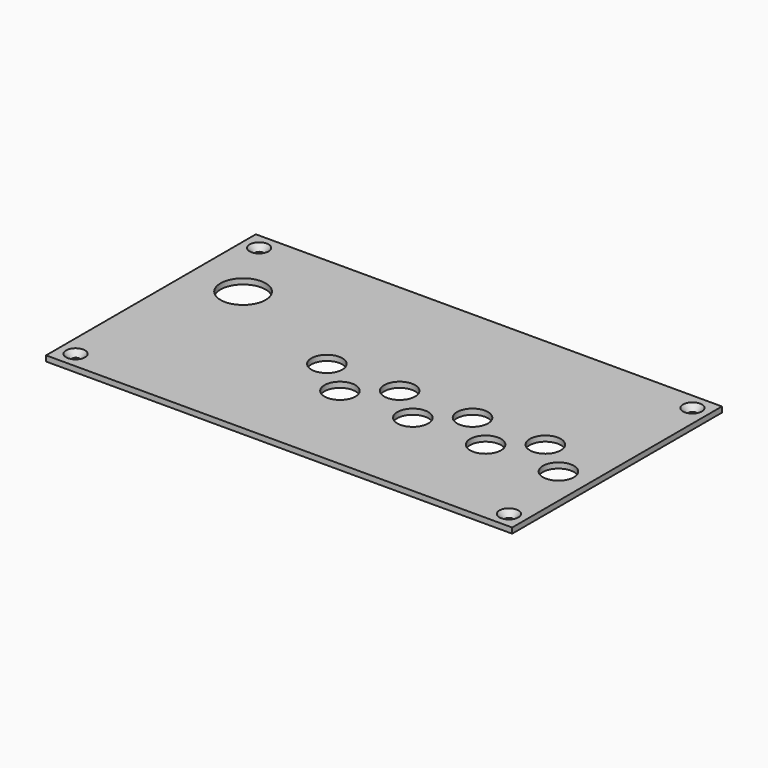
from build123d import *

# Parameters (mm, degrees)
F0_W     = 406.4
F0_H     = 228.6
F0_W_2   = 396.875
F0_H_2   = 219.075
F0_R     = 3.175
F0_R_2   = 13.49375
F0_R_3   = 19.685
F1_DEPTH = 4.7752


# Not quite as in the source:
# - a fillet or chamfer that OpenCascade refuses, or shapes differently, is made with other operations: its cross-section is extruded or revolved along the edge and cut away or added


with BuildPart() as f1:
    # F0 (on Top) → F1 (new body)
    with BuildSketch(Plane.XY):
        with Locations((-26.3652, 4.7498)):
            Rectangle(F0_W, F0_H)
        with Locations((-26.3525, 4.7625)):
            Rectangle(F0_W_2, F0_H_2, mode=Mode.SUBTRACT)
        with Locations((-26.3525, 4.7625)):
            Rectangle(F0_W_2, F0_H_2)
        with Locations((-215.265, -95.25)):
            Circle(F0_R, mode=Mode.SUBTRACT)
        with Locations((-40.64, -25.4)):
            Circle(F0_R_2, mode=Mode.SUBTRACT)
        with Locations((-72.39, 0)):
            Circle(F0_R_2, mode=Mode.SUBTRACT)
        with Locations((162.56, -95.25)):
            Circle(F0_R, mode=Mode.SUBTRACT)
        with Locations((22.86, -25.4)):
            Circle(F0_R_2, mode=Mode.SUBTRACT)
        with Locations((-8.89, 0)):
            Circle(F0_R_2, mode=Mode.SUBTRACT)
        with Locations((54.61, 0)):
            Circle(F0_R_2, mode=Mode.SUBTRACT)
        with Locations((86.36, -25.4)):
            Circle(F0_R_2, mode=Mode.SUBTRACT)
        with Locations((149.86, -25.4)):
            Circle(F0_R_2, mode=Mode.SUBTRACT)
        with Locations((118.11, 0)):
            Circle(F0_R_2, mode=Mode.SUBTRACT)
        with Locations((-183.515, 47.625)):
            Circle(F0_R_3, mode=Mode.SUBTRACT)
        with Locations((-215.265, 104.775)):
            Circle(F0_R, mode=Mode.SUBTRACT)
        with Locations((162.56, 104.775)):
            Circle(F0_R, mode=Mode.SUBTRACT)
    extrude(amount=F1_DEPTH)

    # F2: chamfer of 5.08 on 4 edges, made by hand

    # F2_s1 → F2_t2 (revolve, cut)
    with BuildSketch(Plane.XZ.offset(95.25)):
        Polygon((-212.09, -0.3048), (-207.01, 4.7752), (-212.09, 4.7752), align=None)
    revolve(axis=Axis((-215.265, -95.25, 4.7752), (0, 0, 1)), mode=Mode.SUBTRACT)

    # F2_s3 → F2_t4 (revolve, cut)
    with BuildSketch(Plane.XZ.offset(-104.775)):
        Polygon((-212.09, -0.3048), (-207.01, 4.7752), (-212.09, 4.7752), align=None)
    revolve(axis=Axis((-215.265, 104.775, 4.7752), (0, 0, 1)), mode=Mode.SUBTRACT)

    # F2_s5 → F2_t6 (revolve, cut)
    with BuildSketch(Plane.XZ.offset(-104.775)):
        Polygon((165.735, -0.3048), (170.815, 4.7752), (165.735, 4.7752), align=None)
    revolve(axis=Axis((162.56, 104.775, 4.7752), (0, 0, 1)), mode=Mode.SUBTRACT)

    # F2_s7 → F2_t8 (revolve, cut)
    with BuildSketch(Plane.XZ.offset(95.25)):
        Polygon((165.735, -0.3048), (170.815, 4.7752), (165.735, 4.7752), align=None)
    revolve(axis=Axis((162.56, -95.25, 4.7752), (0, 0, 1)), mode=Mode.SUBTRACT)


solid = f1.part
